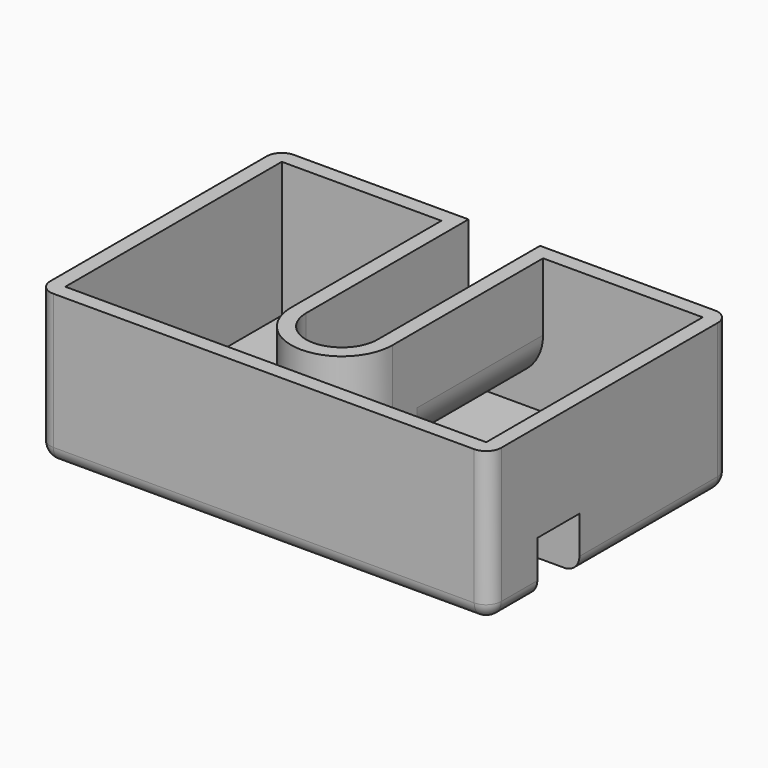
from build123d import *

# Parameters (mm, degrees)
F0_W        = 76.2
F0_H        = 50.8
F2_DEPTH    = 25.4
F1_W        = 76.2
F1_H        = 8.89
F3_DEPTH    = 8.89
F4_R        = 2.54
F6_DEPTH    = 16.51
F7_R        = 5.08
F8_T        = 2.54
F8_T3_DEPTH = 10.16
F8_T5_DEPTH = 37.1348
F8_T7_DEPTH = 37.1348
F8_T9_DEPTH = 81.28


# Not quite as in the source:
# - a shell that OpenCascade refuses in one call is made with other operations: the cavity is built on its own and cut out


with BuildPart() as f2:
    # F0 (on Top) → F2 (new body)
    with BuildSketch(Plane.XY):
        Rectangle(F0_W, F0_H)
    extrude(amount=F2_DEPTH)

    # F1 (on face) → F3 (cut)
    with BuildSketch(Plane.XY):
        with Locations((0, -10.795)):
            Rectangle(F1_W, F1_H)
    extrude(amount=F3_DEPTH, mode=Mode.SUBTRACT)

    # F4
    f4_edges = [f2.edges().sort_by_distance(p)[0] for p in [
        (-38.1, 9.525, 0),
        (0, 25.4, 0),
        (38.1, 9.525, 0),
        (-38.1, -20.32, 0),
        (0, -25.4, 0),
        (38.1, -20.32, 0),
        (-38.1, 25.4, 12.7),
        (-38.1, -25.4, 12.7),
        (38.1, -25.4, 12.7),
        (38.1, 25.4, 12.7),
    ]]
    fillet(f4_edges, radius=F4_R)

    # F5 (on face) → F6 (cut, through all)
    with BuildSketch(Plane.XY.offset(25.4)):
        Polygon((6.0452, 25.4), (-6.0452, 25.4), (-6.0452, -6.35), (-6.0452, -8.89), (6.0452, -8.89), (6.0452, -6.35), align=None)
        with BuildLine():
            Line((6.0452, -8.89), (-6.0452, -8.89))
            ThreePointArc((-6.0452, -8.89), (0, -14.9352), (6.0452, -8.89))
        make_face()
    extrude(amount=-F6_DEPTH, mode=Mode.SUBTRACT)

    # F7
    f7_edges = [f2.edges().sort_by_distance(p)[0] for p in [
        (-6.0452, 9.525, 8.89),
        (6.0452, 9.525, 8.89),
    ]]
    fillet(f7_edges, radius=F7_R)

    # F8: shell of thickness 2.54, made by hand


with BuildPart() as f8_core1:
    # F8_t2: copy of F2
    add(f2.part)

    # the walls: a layer under each face that stays
    f8_faces = [f8_core1.faces().sort_by_distance(p)[0] for p in [
        (23.7066666667, 25.4, 21.59),
        (-6.0452, 8.255, 17.145),
        (-4.5573024484, 9.525, 10.3778975516),
        (0, 9.525, 8.89),
        (4.5573024484, 9.525, 10.3778975516),
        (6.0452, 8.255, 17.145),
        (0, -6.35, 6.985),
        (0, -14.9352, 17.145),
        (-25.4, -13.7583333333, 8.89),
        (38.1, 0, 13.97),
        (0, -25.4, 13.97),
        (-38.1, 0, 13.97),
        (0, 8.255, 0),
        (0, -15.24, 4.445),
        (0, -19.05, 0),
    ]]
    thicken(f8_faces, amount=-F8_T, mode=Mode.SUBTRACT)

    # F8_s4 → F8_t3 (cut)
    with BuildSketch(Plane.XY.offset(6.35)):
        Polygon((-6.0198, -6.3754), (-8.5852, -6.35), (-8.5852, -3.81), (-6.0452, -3.81), align=None)
        Polygon((6.0198, -6.3754), (8.5852, -6.35), (8.5852, -3.81), (6.0452, -3.81), align=None)
    extrude(amount=F8_T3_DEPTH, mode=Mode.SUBTRACT)

    # F8_s6 → F8_t5 (cut)
    with BuildSketch(Plane.YZ.offset(3.5052)):
        Polygon((-6.3754, 8.8646), (-3.81, 8.89), (-3.81, 11.43), (-6.35, 11.43), align=None)
    extrude(amount=F8_T5_DEPTH, mode=Mode.SUBTRACT)

    # F8_s8 → F8_t7 (cut)
    with BuildSketch(Plane.YZ.offset(-40.64)):
        Polygon((-6.3754, 8.8646), (-3.81, 8.89), (-3.81, 11.43), (-6.35, 11.43), align=None)
    extrude(amount=F8_T7_DEPTH, mode=Mode.SUBTRACT)

    # F8_s10 → F8_t9 (cut)
    with BuildSketch(Plane.YZ.offset(-40.64)):
        Polygon((-15.2146, 8.8646), (-15.24, 11.43), (-17.78, 11.43), (-17.78, 8.89), align=None)
    extrude(amount=F8_T9_DEPTH, mode=Mode.SUBTRACT)


with BuildPart() as f2_1:
    add(f2.part)

    # what is left inside the walls is the cavity
    f8_cavity = [f8_core1.part.solids().sort_by_distance(p)[0] for p in [
        (-17.78, 7.62, 25.3746),
    ]]
    add(f8_cavity, mode=Mode.SUBTRACT)


solid = f2_1.part
